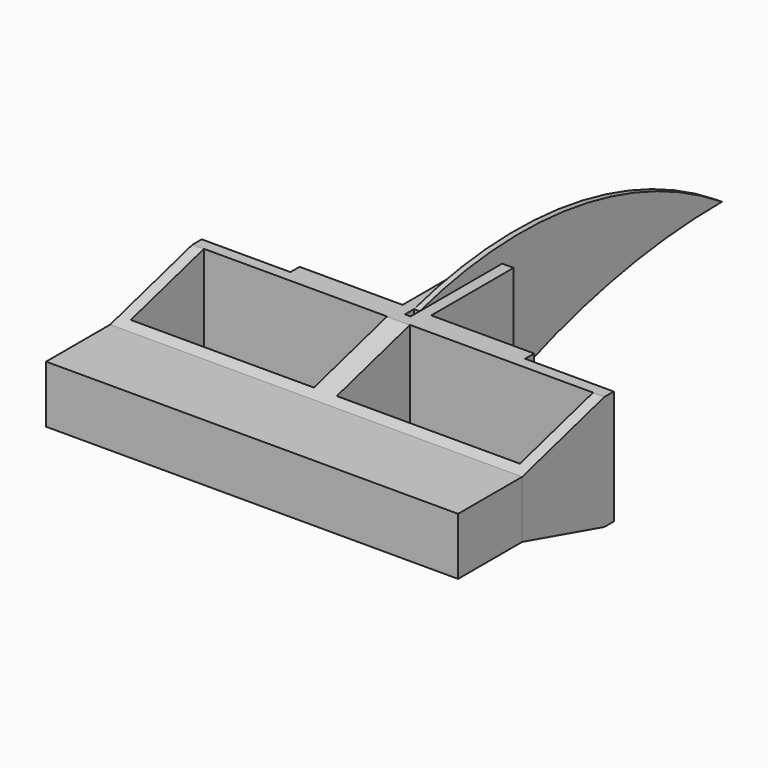
from build123d import *

# Parameters (mm, degrees)
F0_W          = 50.8
F0_H          = 25.4
F1_DEPTH      = 15.875
F1_DEPTH_BACK = 15.875
F2_DEPTH      = 7.9502
F2_DEPTH_BACK = 7.9502
F3_DEPTH      = 15.875
F3_DEPTH_BACK = 15.875
F7_DEPTH      = 57.15
F7_DEPTH_BACK = 57.15
F9_DEPTH      = 0.79375
F9_DEPTH_BACK = 0.79375


# Not quite as in the source:
# - the program builds the solid bodies; features that only make, move or delete a surface that nothing else refers to are left out


with BuildPart() as f1:
    # F0 (on Top) → F1 (new body, two sides)
    with BuildSketch(Plane.XY) as f1_sk:
        Polygon((-57.15, -3.175), (0, -3.175), (57.15, -3.175), (57.15, 28.575), (32.54375, 28.575), (0.79375, 28.575), (-0.79375, 28.575), (-32.54375, 28.575), (-57.15, 28.575), align=None)
        with Locations((-28.575, 12.7)):
            Rectangle(F0_W, F0_H, mode=Mode.SUBTRACT)
        with Locations((28.575, 12.7)):
            Rectangle(F0_W, F0_H, mode=Mode.SUBTRACT)
    extrude(amount=F1_DEPTH)
    extrude(f1_sk.sketch, amount=-F1_DEPTH_BACK)

    # F0 (on Top) → F3 (join, two sides)
    with BuildSketch(Plane.XY) as f3_sk:
        Polygon((-32.54375, 31.75), (-32.54375, 28.575), (-0.79375, 28.575), (-0.79375, 60.325), (-3.96875, 60.325), (-3.96875, 31.75), align=None)
        Polygon((0.79375, 28.575), (32.54375, 28.575), (32.54375, 31.75), (3.96875, 31.75), (3.96875, 60.325), (0.79375, 60.325), align=None)
    extrude(amount=F3_DEPTH)
    extrude(f3_sk.sketch, amount=-F3_DEPTH_BACK)

    # F6 (on Right) → F7 (cut, two sides)
    with BuildSketch(Plane.YZ) as f7_sk:
        Polygon((25.4, -15.9004), (-3.175, -7.9502), (-3.175, -15.9004), align=None)
        Polygon((-3.175, 15.9004), (-3.175, 7.9502), (25.4, 15.9004), align=None)
    extrude(amount=-F7_DEPTH, mode=Mode.SUBTRACT)
    extrude(f7_sk.sketch, amount=F7_DEPTH_BACK, mode=Mode.SUBTRACT)


with BuildPart() as f2:
    # F0 (on Top) → F2 (new body, two sides)
    with BuildSketch(Plane.XY) as f2_sk:
        Polygon((57.15, -3.175), (0, -3.175), (-57.15, -3.175), (-57.15, -25.4), (57.15, -25.4), align=None)
    extrude(amount=F2_DEPTH)
    extrude(f2_sk.sketch, amount=-F2_DEPTH_BACK)


with BuildPart() as f9:
    # F8 (on Right) → F9 (new body, two sides)
    with BuildSketch(Plane.YZ) as f9_sk:
        with BuildLine():
            ThreePointArc((60.325, -15.875), (97.606959116, -4.0109037567), (136.525, 0))
            ThreePointArc((136.525, 0), (85.8723958548, 19.3878126418), (31.75, 15.875))
            Line((31.75, 15.875), (31.75, -15.875))
            Line((31.75, -15.875), (60.325, -15.875))
        make_face()
    extrude(amount=F9_DEPTH)
    extrude(f9_sk.sketch, amount=-F9_DEPTH_BACK)


solid = Compound([f1.part, f2.part, f9.part])
